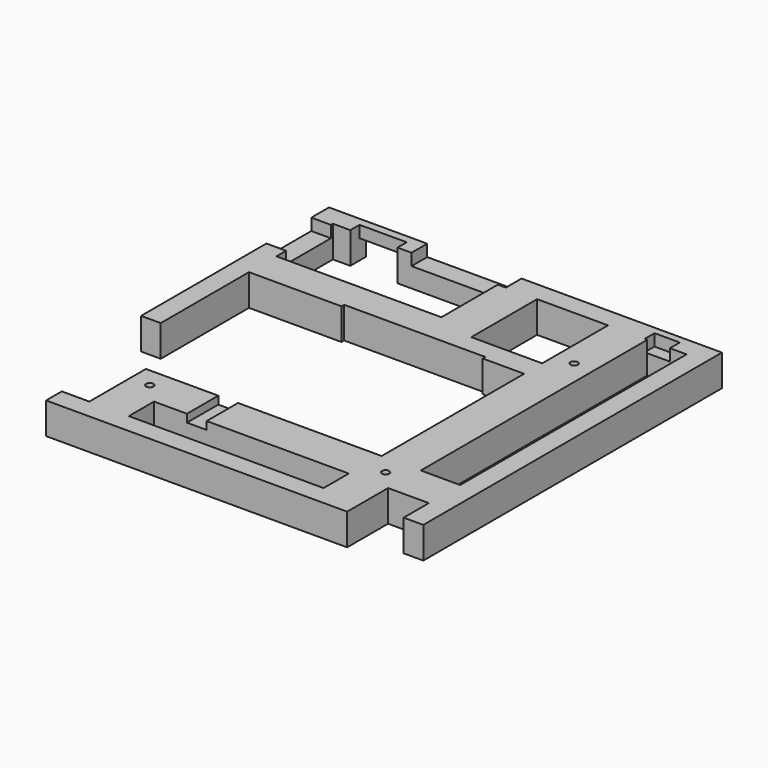
from build123d import *

# Parameters (mm, degrees)
F1_W      = 126.9999492
F1_H      = 127.0000508
F2_DEPTH  = 10.16
F3_W      = 114.2999492
F3_H      = 114.3000508
F4_DEPTH  = 10.161
F5_W      = 10.4391968
F5_H      = 51.0824988
F5_W_2    = 15.240254
F5_H_2    = 6.35
F5_W_3    = 19.531076
F6_DEPTH  = 10.161
F7_W      = 6.3186603262
F7_H      = 12.6597918
F8_DEPTH  = 10.16
F10_D     = 2.3749
F11_R     = 1.18745
F12_DEPTH = 2.794
F15_W     = 12.7
F15_H     = 26.589482
F16_DEPTH = 10.16
F15_H_2   = 10.1803962
F18_D     = 3.4544
F18_DEPTH = 6.35
F18_TIP   = 1.0378064612
F9_W      = 6.35
F9_H      = 18.117566
F9_W_2    = 30.48
F9_H_2    = 6.35
F9_W_3    = 8.1742328233
F9_H_3    = 3.990848
F19_DEPTH = 3.81
F20_W     = 45.6544562851
F20_H     = 1.059942
F21_DEPTH = 10.161
F22_W     = 53.3058220283
F22_H     = 3.769614
F22_W_2   = 15.240254
F22_H_2   = 2.629916
F23_DEPTH = 3.81
F24_W     = 6.379972
F24_H     = 12.6597918
F25_DEPTH = 2.54


# Not quite as in the source:
# - a feature names something its author has since deleted; it is built from what else it names


with BuildPart() as f2:
    # F1 (on Top) → F2 (new body)
    with BuildSketch(Plane.XY):
        with Locations((0.1398778, 0)):
            Rectangle(F1_W, F1_H)
    extrude(amount=-F2_DEPTH)

    # F3 (on face) → F4 (cut, through all)
    with BuildSketch(Plane(origin=(0, 0, -10.16), x_dir=(1, 0, 0), z_dir=(0, 0, -1))):
        with Locations((0.1398778, 0)):
            Rectangle(F3_W, F3_H)
    extrude(amount=-F4_DEPTH, mode=Mode.SUBTRACT)

    # F5 (on face) → F6 (cut, through all)
    with BuildSketch(Plane(origin=(0, 0, -10.16), x_dir=(1, 0, 0), z_dir=(0, 0, -1))):
        with Locations((-58.420254, 37.958776)):
            Rectangle(F5_W, F5_H)
        with Locations((-43.7761126, -60.3250254)):
            Rectangle(F5_W_2, F5_H_2)
        with Locations((53.8743144, 60.3250254)):
            Rectangle(F5_W_3, F5_H_2)
    extrude(amount=-F6_DEPTH, mode=Mode.SUBTRACT)


with BuildPart() as f8:
    # F7 (on face) → F8 (new body)
    with BuildSketch(Plane(origin=(0, 0, -10.16), x_dir=(1, 0, 0), z_dir=(0, 0, -1))):
        Polygon((-37.8689406421, 34.3098374), (-37.8689406421, 46.9696292), (-31.5502803159, 46.9696292), (-31.5502803159, 57.1500254), (-44.2886084, 57.1500254), (-44.2886084, 34.3098374), align=None)
        with Locations((-34.709610479, 40.6397333)):
            Rectangle(F7_W, F7_H)
        Polygon((57.2898524, 46.9696292), (-31.5502803159, 46.9696292), (-31.5502803159, 34.3098374), (31.9114424, 34.3098374), (44.5713104, 34.3098374), (57.2898524, 34.3098374), align=None)
        Polygon((44.5713104, 34.3098374), (31.9114424, 34.3098374), (31.9114424, -23.2499154), (31.9114424, -29.2427535486), (31.9114424, -30.5605434), (31.9114424, -41.8902134), (31.9114424, -57.1500254), (44.5713104, -57.1500254), align=None)
        Polygon((31.9114424, -29.2427535486), (31.9114424, -23.2499154), (-57.0100968, -23.2499154), (-57.0100968, -30.5605434), (31.9114424, -30.5605434), align=None)
    extrude(amount=-F8_DEPTH)

    # F10 (through all)
    with Locations(Plane.XY):
        with Locations((38.2398524, 35.5602794), (38.2398524, -40.639746), (-37.9601476, -40.639746)):
            Hole(F10_D / 2)

    # F11 (on face) → F12 (cut)
    with BuildSketch(Plane(origin=(0, 0, -10.16), x_dir=(1, 0, 0), z_dir=(0, 0, -1))):
        Polygon((-34.2943619493, 40.693121057), (-36.17347893, 43.8410970268), (-39.8392645806, 43.7877219698), (-41.6259332507, 40.586370943), (-39.74681627, 37.4383949732), (-36.0810306194, 37.4917700302), align=None)
        with Locations((-37.9601476, 40.639746)):
            Circle(F11_R, mode=Mode.SUBTRACT)
        Polygon((34.5740667493, 40.586370943), (36.45318373, 37.4383949732), (40.1189693806, 37.4917700302), (41.9056380507, 40.693121057), (40.02652107, 43.8410970268), (36.3607354194, 43.7877219698), align=None)
        Polygon((36.3607354194, -32.4123034302), (34.5740667493, -35.613654457), (36.45318373, -38.7616304268), (40.1189693806, -38.7082553698), (41.9056380507, -35.506904343), (40.02652107, -32.3589283732), align=None)
    extrude(amount=-F12_DEPTH, mode=Mode.SUBTRACT)

    # F14: union F2
    add(f2.part)


with BuildPart() as f16:
    # F15 (on face) → F16 (new body, through all)
    with BuildSketch(Plane.XY):
        with Locations((2.6457252283, 43.8552844)):
            Rectangle(F15_W, F15_H)
    extrude(amount=-F16_DEPTH)


with BuildPart() as f16b:
    # F15 (on face) → F16, piece 2 (new body, through all)
    with BuildSketch(Plane.XY):
        with Locations((37.7587764, -52.0598273)):
            Rectangle(F15_W, F15_H_2)
    extrude(amount=-F16_DEPTH)


with BuildPart() as f16_1:
    add(f16.part)

    # F17: union F16b, F8
    add(f16b.part)
    add(f8.part)

    # F18
    with Locations(Plane(origin=(0, 0, -10.16), x_dir=(1, 0, 0), z_dir=(0, 0, -1))):
        with Locations((0.1805810421, 40.6397333), (-4.5459396, 60.3250254), (-60.1850968, -25.6824734), (38.2398524, -60.3250254), (60.4648524, -38.1000254), (60.4648524, 31.7500254)):
            Hole(F18_D / 2, depth=F18_DEPTH)
            with Locations((0, 0, -(F18_DEPTH + F18_TIP / 2))):  # 118° drill point
                Cone(0, F18_D / 2, F18_TIP, mode=Mode.SUBTRACT)

    # F9 (on face) → F19 (cut)
    with BuildSketch(Plane.XY):
        with Locations((-60.1850968, 47.2840304)):
            Rectangle(F9_W, F9_H)
        with Locations((-16.3704016, 60.3250254)):
            Rectangle(F9_W_2, F9_H_2)
        with Locations((47.8253068116, 59.1454494)):
            Rectangle(F9_W_3, F9_H_3)
    extrude(amount=-F19_DEPTH, mode=Mode.SUBTRACT)

    # F20 (on face) → F21 (cut, through all)
    with BuildSketch(Plane.XY):
        with Locations((-4.2932037426, 23.7798864)):
            Rectangle(F20_W, F20_H)
    extrude(amount=-F21_DEPTH, mode=Mode.SUBTRACT)

    # F22 (on face) → F23 (join)
    with BuildSketch(Plane.XY):
        with Locations((-30.3571857859, 32.4453504)):
            Rectangle(F22_W, F22_H)
        with Locations((-43.7761126, 62.1850674)):
            Rectangle(F22_W_2, F22_H_2)
    extrude(amount=-F23_DEPTH)

    # F24 (on face) → F25 (cut)
    with BuildSketch(Plane.XY):
        with Locations((-17.7036476, -40.6397333)):
            Rectangle(F24_W, F24_H)
    extrude(amount=-F25_DEPTH, mode=Mode.SUBTRACT)


solid = f16_1.part
